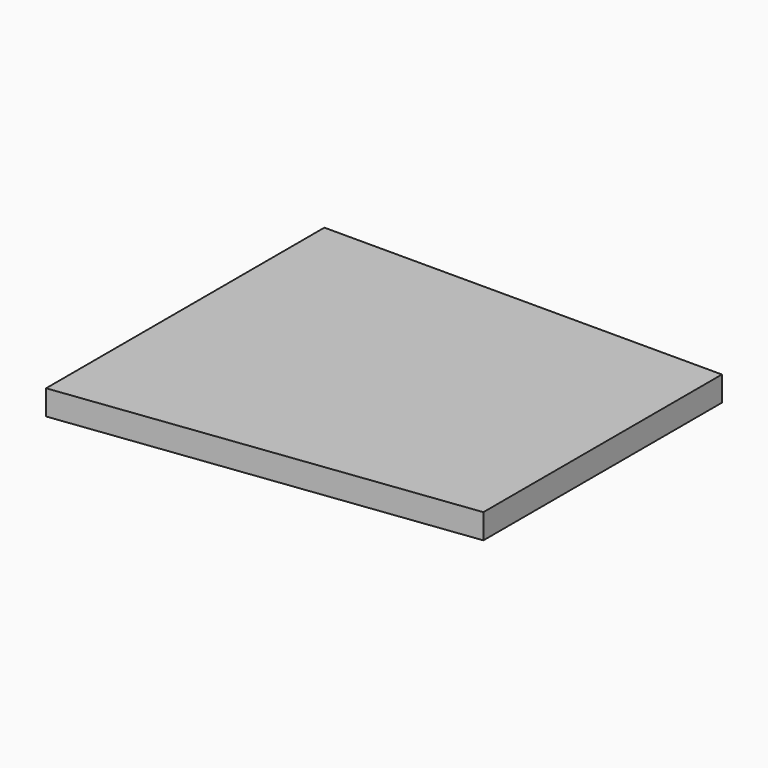
from build123d import *

# Parameters (mm, degrees)
F1_DEPTH     = 3.175
F2_TEXT_SIZE = 7.2190220012
F3_DEPTH     = 0.0762
F4_TEXT_SIZE = 4.1546759247
F5_DEPTH     = 0.0762


# Not quite as in the source:
# - Text() gives the source's letters only with a copy of the font that has no kerning and outlines rounded to 1/6400 em; it was checked with that copy


with BuildPart() as f1:
    # F0 (on Top) → F1 (new body)
    with BuildSketch(Plane.XY):
        Polygon((-6.35, -3.175), (-57.15, -3.175), (-57.15, -47.625), (-6.35, -41.275), align=None)
    extrude(amount=F1_DEPTH)

    # F2 (on face) → F3 (cut)
    with BuildSketch(Plane.XY.offset(3.175)):
        with Locations((-22.3182930972, 11.9338437947)):
            Text('Plead the 2nd', F2_TEXT_SIZE, font='Open Sans', font_style=FontStyle.ITALIC, text_align=(TextAlign.LEFT, TextAlign.BOTTOM))
    extrude(amount=-F3_DEPTH, mode=Mode.SUBTRACT)

    # F4 (on face) → F5 (cut)
    with BuildSketch(Plane.XY.offset(3.175)):
        with Locations((12.8858890384, 4.7171539627)):
            Text('001', F4_TEXT_SIZE, font='Open Sans', font_style=FontStyle.ITALIC, text_align=(TextAlign.LEFT, TextAlign.BOTTOM))
    extrude(amount=-F5_DEPTH, mode=Mode.SUBTRACT)


solid = f1.part
